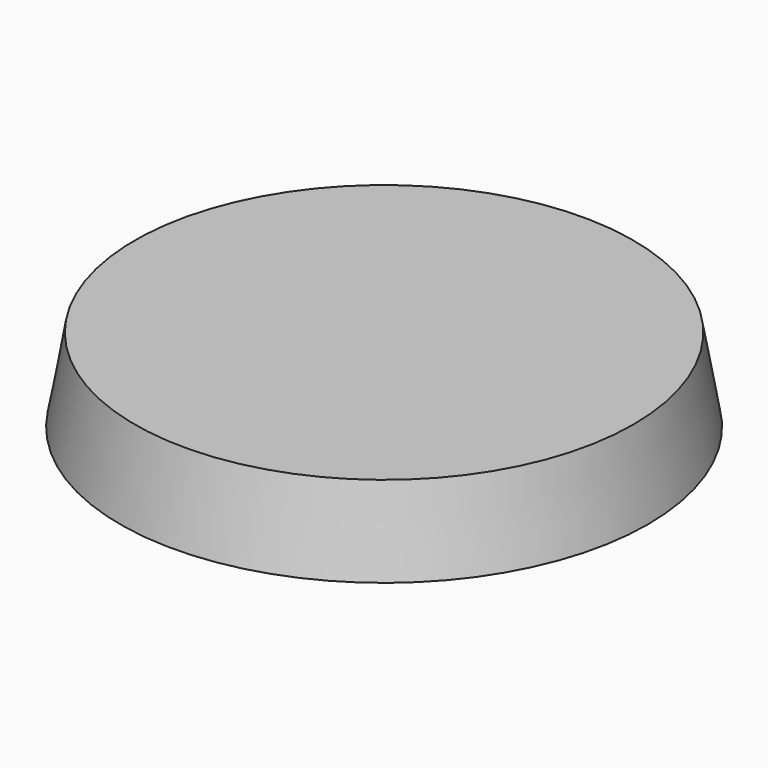
from build123d import *

# Parameters (mm, degrees)
F0_R         = 30
F1_DEPTH     = 10
F1_TAPER     = -10
F2_TEXT_SIZE = 14.4150047094
F3_DEPTH     = 1


# Not quite as in the source:
# - Text() gives the source's letters only with a copy of the font that has no kerning and outlines rounded to 1/6400 em; it was checked with that copy


with BuildPart() as f1:
    # F0 (on Top) → F1 (new body)
    with BuildSketch(Plane.XY):
        Circle(F0_R)
    extrude(amount=-F1_DEPTH, taper=F1_TAPER)

    # F2 (on face) → F3 (cut)
    with BuildSketch(Plane(origin=(0, 0, -10), x_dir=(1, 0, 0), z_dir=(0, 0, -1))):
        with Locations((-26, -4.6667001882)):
            Text('Amanda', F2_TEXT_SIZE, font='Open Sans', font_style=FontStyle.ITALIC, text_align=(TextAlign.LEFT, TextAlign.BOTTOM))
    extrude(amount=-F3_DEPTH, mode=Mode.SUBTRACT)


solid = f1.part
